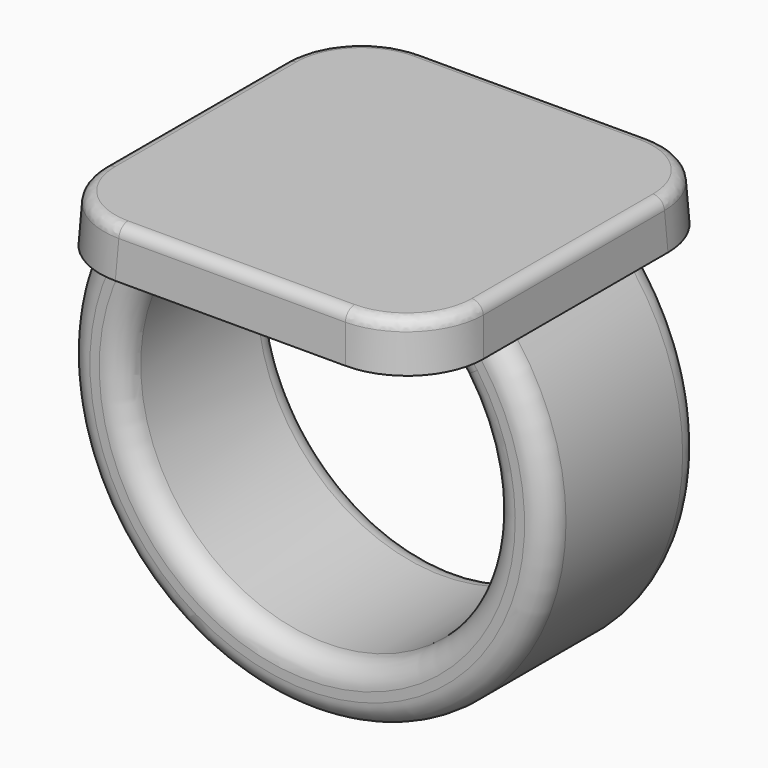
from build123d import *

# Parameters (mm, degrees)
F0_W          = 25.4
F0_H          = 25.4
F1_DEPTH      = 3.175
F1_TAPER      = 3
F3_W          = 5.08
F3_H          = 12.7
F6_DEPTH      = 6.35
F6_DEPTH_BACK = 6.35
F7_R          = 5.08
F8_R          = 1.524
F9_R          = 0.762


with BuildPart() as f1:
    # F0 (on Top) → F1 (new body)
    with BuildSketch(Plane.XY):
        Rectangle(F0_W, F0_H)
    extrude(amount=F1_DEPTH, taper=F1_TAPER)

    # F4: sweep along a path in F2
    with BuildLine(Plane.XZ) as f4_path:
        ThreePointArc((-10.16, 0), (0, -23.5582897328), (10.16, 0))
    # F3 (on face) → F4 (sweep)
    with BuildSketch(Plane(origin=(0, 0, 0), x_dir=(1, 0, 0), z_dir=(0, 0, -1))):
        with Locations((-10.16, 0)):
            Rectangle(F3_W, F3_H)
    sweep(path=f4_path.line)

    # F5 (on Front) → F6 (join, two sides)
    with BuildSketch(Plane.XZ) as f6_sk:
        with BuildLine():
            ThreePointArc((7.62, 0), (8.9072265211, -1.1822790439), (10.0130578512, -2.535746045))
            Line((10.0130578512, -2.535746045), (10.16, 0))
            Line((10.16, 0), (7.62, 0))
        make_face()
    extrude(amount=F6_DEPTH)
    extrude(f6_sk.sketch, amount=-F6_DEPTH_BACK)

    # F7
    f7_edges = [f1.edges().sort_by_distance(p)[0] for p in [
        (-12.616803, 12.616803, 1.5875),
        (-12.616803, -12.616803, 1.5875),
        (12.616803, -12.616803, 1.5875),
        (12.616803, 12.616803, 1.5875),
    ]]
    fillet(f7_edges, radius=F7_R)

    # F8
    f8_edges = [f1.edges().sort_by_distance(p)[0] for p in [
        (-1.743325, -6.35, -21.711017),
        (8.907227, -6.35, -1.182279),
        (-1.743325, 6.35, -21.711017),
        (0, -6.35, -25.501344),
        (0, 6.35, -25.501344),
        (8.907227, 6.35, -1.182279),
    ]]
    fillet(f8_edges, radius=F8_R)

    # F9
    f9_edges = [f1.edges().sort_by_distance(p)[0] for p in [
        (12.533605, 0, 3.175),
        (11.048589, -11.048589, 3.175),
        (11.048589, 11.048589, 3.175),
        (0, -12.533605, 3.175),
        (0, 12.533605, 3.175),
        (-11.048589, -11.048589, 3.175),
        (-11.048589, 11.048589, 3.175),
        (-12.533605, 0, 3.175),
    ]]
    fillet(f9_edges, radius=F9_R)


solid = f1.part
